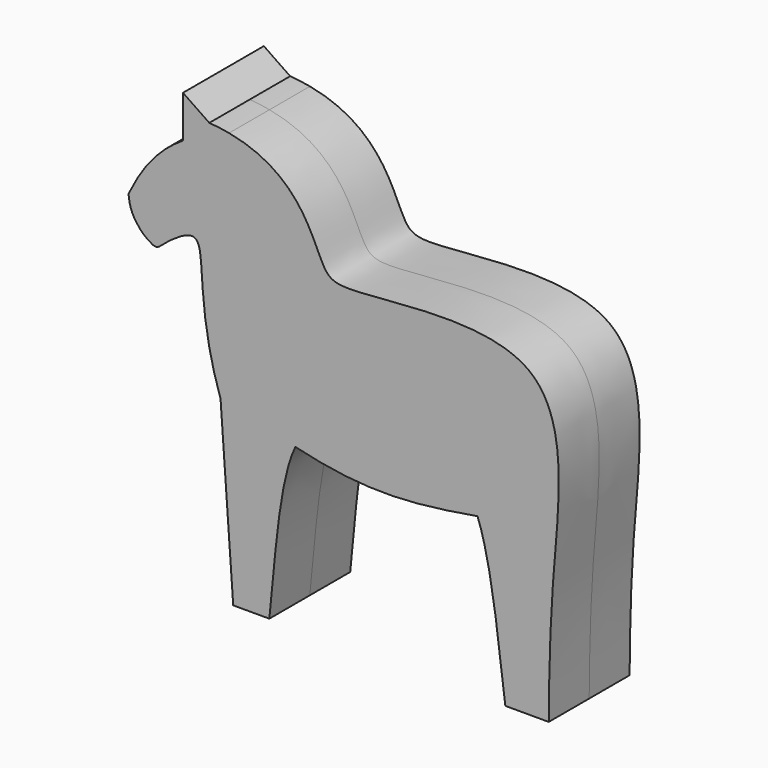
from build123d import *

# Parameters (mm, degrees)
F1_DEPTH = 12.7


with BuildPart() as f1:
    # F0 (on Front) → F1 (new body, symmetric)
    with BuildSketch(Plane.XZ):
        with BuildLine():
            add(Edge.make_bspline(
                [(29.4644571841, -60.1132586598), (27.6855829591, -46.3318706801), (26.0364115238, -29.8171713948), (22.4748793989, -20.4304866493)],
                knots=[0, 0, 0, 0, 40.2936296709, 40.2936296709, 40.2936296709, 40.2936296709], degree=3))
            Line((29.4644571841, -60.1132586598), (40.3708852828, -60.1132586598))
            add(Edge.make_bspline(
                [(-39.9478672487, 44.0147390983), (-22.6170819874, 40.7392920594), (-17.6583308267, 21.8449652817), (-10.5823233679, 17.4452892369), (48.2060896937, 28.4705173137), (40.6121053954, -27.0892647533), (40.4531992639, -51.9750322816), (40.3708852828, -60.1132586598)],
                knots=[0.0176141395, 0.0176141395, 0.0176141395, 0.0176141395, 0.2155433835, 0.3127139787, 0.5541696156, 0.7899221691, 1, 1, 1, 1], degree=3))
            add(Edge.make_bspline(
                [(-51.525823772, 38.5839095885), (-48.427228892, 40.5626276502), (-44.6559490871, 42.3665309751), (-39.9478672487, 44.0147390983)],
                knots=[23.1608101494, 23.1608101494, 23.1608101494, 23.1608101494, 33.4552840805, 33.4552840805, 33.4552840805, 33.4552840805], degree=3))
            add(Edge.make_bspline(
                [(-65.2326749397, 22.3562452086), (-62.0634924721, 28.7954880253), (-58.4971336441, 34.1321315111), (-51.525823772, 38.5839095885)],
                knots=[0, 0, 0, 0, 23.1608101494, 23.1608101494, 23.1608101494, 23.1608101494], degree=3))
            add(Edge.make_bspline(
                [(-65.2326749397, 22.3562452086), (-64.9142132763, 19.1417994226), (-63.1920002018, 16.5369528749), (-61.4708318004, 14.3936398975), (-59.2138856774, 13.1071134676)],
                knots=[0, 0, 0, 0, 0.4981667475, 0.9372778592, 0.9372778592, 0.9372778592, 0.9372778592], degree=3))
            ThreePointArc((-59.2138856774, 13.1071134676), (-58.2461064449, 12.9092024326), (-57.3486451177, 13.3219112729))
            add(Edge.make_bspline(
                [(-57.3486451177, 13.3219112729), (-55.1020312441, 15.4039535235), (-43.1513826069, 24.2493514779), (-49.0148457206, 5.0786043936), (-42.0894920826, -15.4795860872)],
                knots=[0.0422614145, 0.0422614145, 0.0422614145, 0.0422614145, 0.3570922222, 1, 1, 1, 1], degree=3))
            Line((-42.0894920826, -15.4795860872), (-38.9069225571, -60.1132586598))
            Line((-38.9069225571, -60.1132586598), (-29.8342294991, -60.1132586598))
            add(Edge.make_bspline(
                [(-29.8342294991, -60.1132586598), (-28.3491642525, -46.4075747877), (-27.4474639446, -28.6016501486), (-23.295590654, -19.9795458466)],
                knots=[0, 0, 0, 0, 40.6628663786, 40.6628663786, 40.6628663786, 40.6628663786], degree=3))
            add(Edge.make_bspline(
                [(-23.295590654, -19.9795458466), (-5.7089058682, -24.2634825408), (5.3391372785, -23.3616009355), (22.4748793989, -20.4304866493)],
                knots=[0, 0, 0, 0, 45.7726913834, 45.7726913834, 45.7726913834, 45.7726913834], degree=3))
        make_face()
        with BuildLine():
            add(Edge.make_bspline(
                [(-51.525823772, 38.5839095885), (-48.427228892, 40.5626276502), (-44.6559490871, 42.3665309751), (-39.9478672487, 44.0147390983)],
                knots=[23.1608101494, 23.1608101494, 23.1608101494, 23.1608101494, 33.4552840805, 33.4552840805, 33.4552840805, 33.4552840805], degree=3))
            add(Edge.make_bspline(
                [(-44.9170466202, 44.6540898628), (-43.143386035, 44.5232937495), (-41.4901702624, 44.306228016), (-39.9478672487, 44.0147390983)],
                knots=[0, 0, 0, 0, 0.0176141395, 0.0176141395, 0.0176141395, 0.0176141395], degree=3))
            Line((-44.9170466202, 44.6540898628), (-51.525823772, 49.1643957794))
            Line((-51.525823772, 49.1643957794), (-51.525823772, 38.5839095885))
        make_face()
    extrude(amount=F1_DEPTH, both=True)


solid = f1.part
